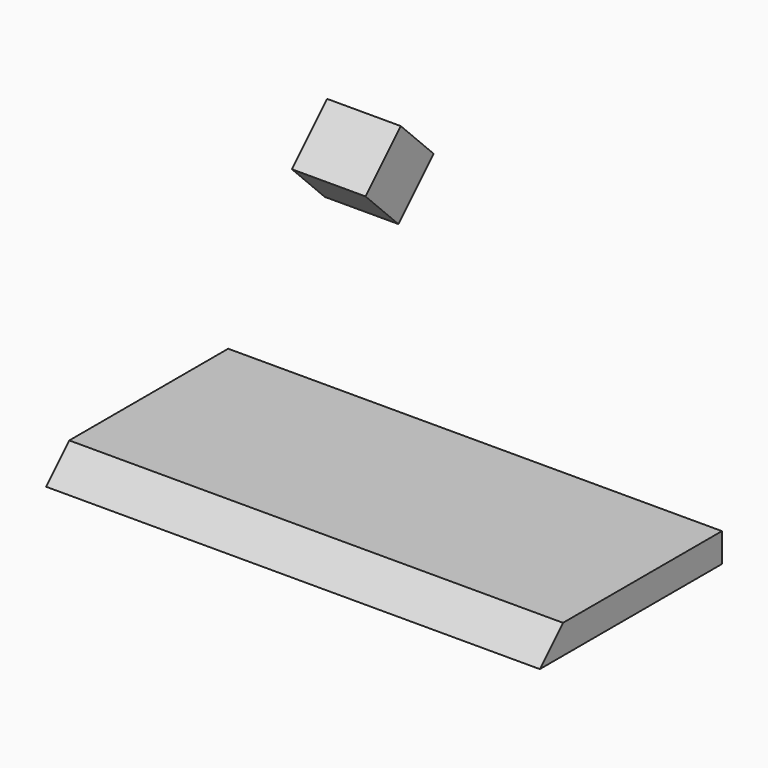
from build123d import *

# Parameters (mm, degrees)
F0_W     = 85.1660892367
F0_H     = 39.2623580992
F1_DEPTH = 5
F2_SIZE  = 4.99999
F3_W     = 12.6967811957
F3_H     = 10.7434242964
F4_DEPTH = 10


# Not quite as in the source:
# - a fillet or chamfer is up to 0.001 mm smaller than in the source, because OpenCascade refuses the exact size


with BuildPart() as f1:
    # F0 (on Top) → F1 (new body)
    with BuildSketch(Plane.XY):
        Rectangle(F0_W, F0_H)
    extrude(amount=F1_DEPTH)

    # F2 (size 5 in the source; OpenCascade refuses exactly that, so slightly less here)
    f2_edges = [f1.edges().sort_by_distance(p)[0] for p in [
        (0, -19.631179, 5),
    ]]
    chamfer(f2_edges, length=F2_SIZE)


with BuildPart() as f4:
    # F3 (on face) → F4 (new body)
    with BuildSketch(Plane(origin=(0, -9.8155895248, 9.8155895248), x_dir=(1, 0, 0), z_dir=(0, -0.7071067812, 0.7071067812))):
        with Locations((-16.7988198809, 42.101662606)):
            Rectangle(F3_W, F3_H)
    extrude(amount=F4_DEPTH)


solid = Compound([f1.part, f4.part])
